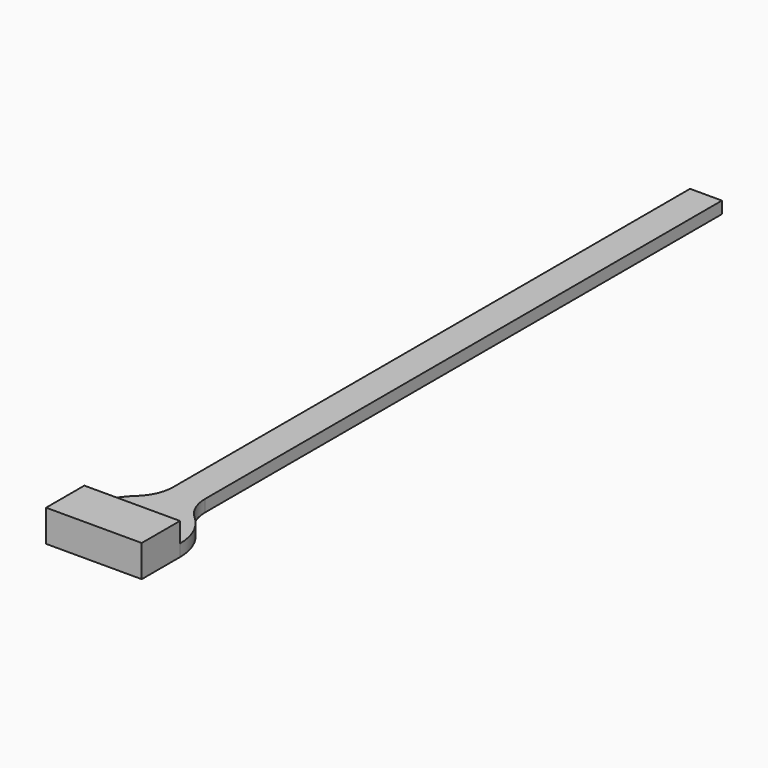
from build123d import *

# Parameters (mm, degrees)
F0_W     = 15.24
F0_H     = 7.62
F1_DEPTH = 5.08
F2_W     = 12.7
F2_H     = 1.905
F3_DEPTH = 5.08
F5_DEPTH = 1.905


# Not quite as in the source:
# - a feature names something its author has since deleted; it is built from what else it names


with BuildPart() as f1:
    # F0 (on Top) → F1 (new body)
    with BuildSketch(Plane.XY):
        with Locations((7.62, 3.81)):
            Rectangle(F0_W, F0_H)
    extrude(amount=F1_DEPTH)

    # F2 (on face) → F3 (cut, through all)
    with BuildSketch(Plane(origin=(0, 7.62, 0), x_dir=(-1, 0, 0), z_dir=(0, 1, 0))):
        with Locations((-7.62, 2.8575)):
            Rectangle(F2_W, F2_H)
    extrude(amount=-F3_DEPTH, mode=Mode.SUBTRACT)

    # F4 (on face) → F5 (join, through all)
    with BuildSketch(Plane(origin=(0, 0, 0), x_dir=(1, 0, 0), z_dir=(0, 0, -1))):
        with BuildLine():
            ThreePointArc((10.16, -18.9792253257), (10.7132695997, -16.3868486813), (12.2766666667, -14.2462147733))
            ThreePointArc((12.2766666667, -14.2462147733), (14.4654225604, -11.2493273022), (15.24, -7.62))
            Line((15.24, -7.62), (7.62, -7.62))
            Line((7.62, -7.62), (7.62, -121.92))
            Line((7.62, -121.92), (10.16, -121.92))
            Line((10.16, -121.92), (10.16, -18.9792253257))
        make_face()
    extrude(amount=-F5_DEPTH)

    # F6: F1 across face


with BuildPart() as f1_1:
    add(f1.part)
    add(f1.part.mirror(Plane(origin=(7.62, 64.77, 0.9525), x_dir=(0, -1, 0), z_dir=(-1, 0, 0))))


solid = f1_1.part
